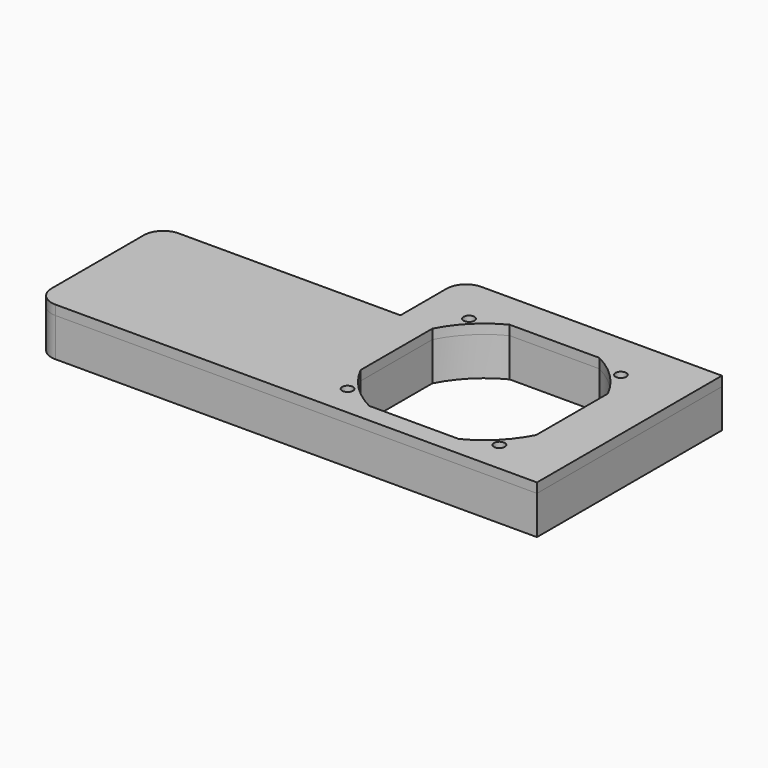
from build123d import *

# Parameters (mm, degrees)
F0_R     = 1.778
F1_DEPTH = 3.175
F2_DEPTH = 12.7


# Not quite as in the source:
# - a length typed as a fraction of an inch, garbled in the dataset ("3 / 203.2 mm" for 3/8 in), is restored
# - a feature names something its author has since deleted; it is built from what else it names


with BuildPart() as f1:
    # F0 (on Top) → F1 (new body)
    with BuildSketch(Plane.XY):
        with BuildLine():
            Line((-113.12525, -35.306), (32.92475, -35.306))
            Line((32.92475, -35.306), (45.6247710268, -35.306))
            Line((45.6247710268, -35.306), (45.6247710268, 40.894))
            Line((45.6247710268, 40.894), (32.92475, 40.894))
            Line((32.92475, 40.894), (-33.6550021708, 40.894))
            ThreePointArc((-33.6550021708, 40.894), (-38.1451302313, 39.0341280605), (-40.0050021708, 34.544))
            Line((-40.0050021708, 34.544), (-40.0050021708, 15.494))
            Line((-40.0050021708, 15.494), (-113.12525, 15.494))
            ThreePointArc((-113.12525, 15.494), (-117.6153780605, 13.6341280605), (-119.47525, 9.144))
            Line((-119.47525, 9.144), (-119.47525, -28.956))
            ThreePointArc((-119.47525, -28.956), (-117.6153780605, -33.4461280605), (-113.12525, -35.306))
        make_face()
        with Locations((-25.019, -25.019)):
            Circle(F0_R, mode=Mode.SUBTRACT)
        with Locations((25.019, -25.019)):
            Circle(F0_R, mode=Mode.SUBTRACT)
        with BuildLine():
            ThreePointArc((-28.956, 14.7844583262), (-22.9894556699, 22.9894556699), (-14.7844583262, 28.956))
            Line((-14.7844583262, 28.956), (14.7844583262, 28.956))
            ThreePointArc((14.7844583262, 28.956), (22.9894556699, 22.9894556699), (28.956, 14.7844583262))
            Line((28.956, 14.7844583262), (28.956, -14.7844583262))
            ThreePointArc((28.956, -14.7844583262), (22.9894556699, -22.9894556699), (14.7844583262, -28.956))
            Line((14.7844583262, -28.956), (-14.7844583262, -28.956))
            ThreePointArc((-14.7844583262, -28.956), (-22.9894556699, -22.9894556699), (-28.956, -14.7844583262))
            Line((-28.956, -14.7844583262), (-28.956, 14.7844583262))
        make_face(mode=Mode.SUBTRACT)
        with Locations((-25.019, 25.019)):
            Circle(F0_R, mode=Mode.SUBTRACT)
        with Locations((25.019, 25.019)):
            Circle(F0_R, mode=Mode.SUBTRACT)
    extrude(amount=-F1_DEPTH)


with BuildPart() as f2:
    # F2 (new): a face of the model
    f2_faces = [f1.part.faces().sort_by_distance(p)[0] for p in [
        (-40.3802916148, -2.9400750607, -3.175),
    ]]
    extrude(f2_faces, amount=F2_DEPTH)


solid = Compound([f1.part, f2.part])
